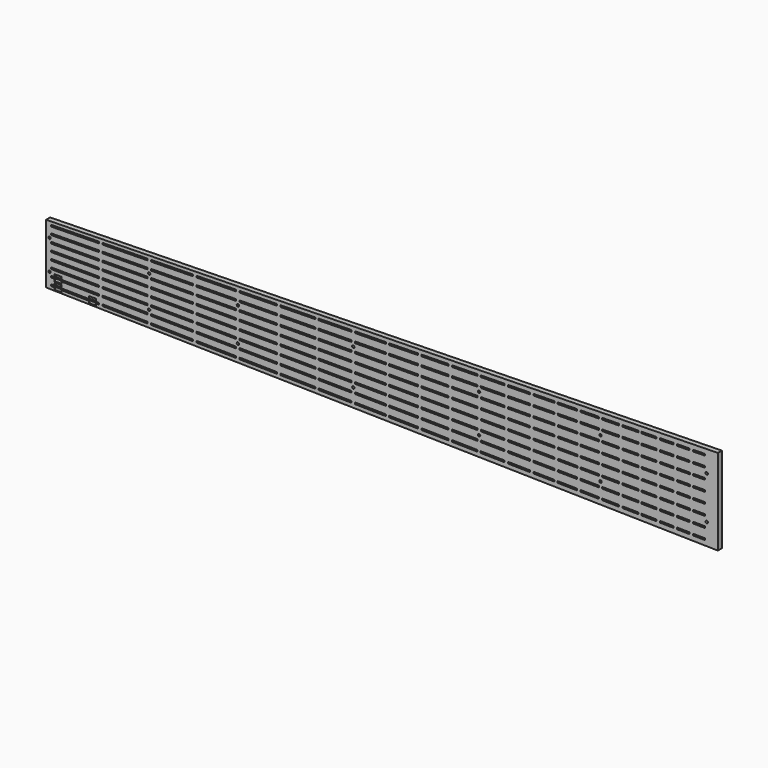
from build123d import *

# Parameters (mm, degrees)
F2_DEPTH  = 4.7625
F4_DEPTH  = 4.7635
F5_R      = 1.1303
F6_DEPTH  = 984
F8_DEPTH  = 4.7635
F9_W      = 6.5
F9_H      = 6.5
F10_DEPTH = 1


# Not quite as in the source:
# - an extrude ends at something that could not be found from the text; its depth is read off the source's solid


with BuildPart() as f2:
    # F1 (on Front) → F2 (new body)
    with BuildSketch(Plane.XZ):
        Polygon((0, 56.388), (0, 0), (635, -12.446), (635, 68.834), align=None)
    extrude(amount=F2_DEPTH)

    # F0 (on Front) → F4 (cut, through all)
    with BuildSketch(Plane.XZ):
        Polygon((4.7746291289, 4.2061348375), (4.7618279084, 3.4442423721), (4.749026688, 2.6823499068), (50.0380481272, 1.9214095194), (50.0508493476, 2.6833019848), (50.0636505681, 3.4451944501), align=None)
        Polygon((53.2382025071, 3.3918560315), (53.2254012866, 2.6299635662), (53.2126000661, 1.8680711009), (95.7808019259, 1.1528455786), (95.7936031464, 1.9147380439), (95.8064043669, 2.6766305093), align=None)
        Polygon((98.9809563058, 2.6232920907), (98.9681550853, 1.8613996253), (98.9553538649, 1.09950716), (138.9572987301, 0.4273995619), (138.9700999505, 1.1892920272), (138.982901171, 1.9511844925), align=None)
        Polygon((142.1574531099, 1.897846074), (142.1446518895, 1.1359536086), (142.131850669, 0.3740611433), (179.7022411275, -0.2571917865), (179.7150423479, 0.5047006789), (179.7278435684, 1.2665931442), align=None)
        Polygon((182.9023955073, 1.2132547257), (182.8895942869, 0.4513622603), (182.8767930664, -0.310530205), (218.1753725717, -0.9036124556), (218.1881737921, -0.1417199903), (218.2009750126, 0.6201724751), align=None)
        Polygon((221.3755269515, 0.5668340565), (221.3627257311, -0.1950584089), (221.3499245106, -0.9569508742), (254.4811739161, -1.5136179197), (254.4939751366, -0.7517254543), (254.506776357, 0.010167011), align=None)
        Polygon((257.681328296, -0.0431714076), (257.6685270755, -0.8050638729), (257.6557258551, -1.5669563382), (288.750030358, -2.0893988941), (288.7628315785, -1.3275064288), (288.775632799, -0.5656139634), align=None)
        Polygon((291.9501847379, -0.618952382), (291.9373835174, -1.3808448473), (291.924582297, -2.1427373127), (321.0950575321, -2.6328559335), (321.1078587526, -1.8709634681), (321.120659973, -1.1090710028), align=None)
        Polygon((324.295211912, -1.1624094214), (324.2824106915, -1.9243018867), (324.2696094711, -2.6861943521), (351.6250536824, -3.1458170521), (351.6378549029, -2.3839245867), (351.6506561233, -1.6220321214), align=None)
        Polygon((354.8252080623, -1.67537054), (354.8124068418, -2.4372630053), (354.7996056214, -3.1991554707), (380.441909228, -3.6299941998), (380.4547104484, -2.8681017344), (380.4675116689, -2.1062092691), align=None)
        Polygon((383.6420636078, -2.1595476876), (383.6292623874, -2.921440153), (383.6164611669, -3.6833326183), (407.6406067628, -4.086983262), (407.6534079833, -3.3250907967), (407.6662092037, -2.5631983313), align=None)
        Polygon((410.8407611427, -2.6165367499), (410.8279599222, -3.3784292152), (410.8151587017, -4.1403216806), (433.3135384465, -4.5183366002), (433.326339667, -3.7564441348), (433.3391408874, -2.9945516695), align=None)
        Polygon((436.5136928264, -3.0478900881), (436.5008916059, -3.8097825534), (436.4880903855, -4.5716750188), (457.5453251356, -4.9254760032), (457.558126356, -4.1635835378), (457.5709275765, -3.4016910725), align=None)
        Polygon((460.7454795155, -3.455029491), (460.732678295, -4.2169219564), (460.7198770745, -4.9788144217), (480.417133774, -5.3097652276), (480.4299349945, -4.5478727623), (480.4427362149, -3.7859802969), align=None)
        Polygon((483.6172881539, -3.8393187155), (483.6044869334, -4.6012111808), (483.591685713, -5.3631036462), (502.004950437, -5.672480982), (502.0177516575, -4.9105885166), (502.0305528779, -4.1486960513), align=None)
        Polygon((505.2051048169, -4.2020344698), (505.1923035964, -4.9639269352), (505.179502376, -5.7258194005), (522.3813072873, -6.0148419423), (522.3941085077, -5.252949477), (522.4069097282, -4.4910570116), align=None)
        Polygon((525.5814616672, -4.5443954302), (525.5686604467, -5.3062878956), (525.5558592262, -6.0681803609), (541.6135556188, -6.3379797367), (541.6263568392, -5.5760872713), (541.6391580597, -4.814194806), align=None)
        Polygon((544.8137099986, -4.8675332245), (544.8009087782, -5.6294256899), (544.7881075577, -6.3913181552), (559.7673197691, -6.6429969767), (559.7801209896, -5.8811045114), (559.79292221, -5.119212046), align=None)
        Polygon((562.967474149, -5.1725504646), (562.9546729285, -5.93444293), (562.9418717081, -6.6963353953), (576.901316251, -6.9308802099), (576.9141174715, -6.1689877446), (576.9269186919, -5.4070952792), align=None)
        Polygon((580.1014706309, -5.4604336978), (580.0886694104, -6.2223261632), (580.07586819, -6.9842186285), (593.0742615771, -7.2026159837), (593.0870627976, -6.4407235183), (593.099864018, -5.678831053), align=None)
        Polygon((596.274415957, -5.7321694715), (596.2616147365, -6.4940619369), (596.2488135161, -7.2559544022), (608.3388279132, -7.4590892889), (608.3516291337, -6.6971968236), (608.3644303541, -5.9353043582), align=None)
        Polygon((611.5389822931, -5.9886427768), (611.5261810726, -6.7505352421), (611.5133798522, -7.5124277075), (622.747687425, -7.7011851168), (622.7604886455, -6.9392926514), (622.773289866, -6.1774001861), align=None)
        Polygon((4.7713008369, 11.2775468317), (4.762157108, 10.5156016944), (4.7530133791, 9.7536565571), (50.0451657853, 9.210127709), (50.0543095142, 9.9720728463), (50.0634532431, 10.7340179835), align=None)
        Polygon((53.2382246484, 10.6959191131), (53.2290809195, 9.9339739759), (53.2199371906, 9.1720288386), (95.7910819189, 8.6611534655), (95.8002256478, 9.4230986028), (95.8093693767, 10.1850437401), align=None)
        Polygon((98.984140782, 10.1469448697), (98.9749970531, 9.3849997324), (98.9658533242, 8.6230545951), (138.9705636448, 8.1429777393), (138.9797073737, 8.9049228766), (138.9888511026, 9.6668680139), align=None)
        Polygon((142.1636225079, 9.6287691434), (142.154478779, 8.8668240062), (142.1453350501, 8.1048788689), (179.7183228632, 7.6539839191), (179.7274665921, 8.4159290563), (179.736610321, 9.1778741936), align=None)
        Polygon((182.9113817264, 9.1397753232), (182.9022379975, 8.3778301859), (182.8930942686, 7.6158850487), (218.1941140714, 7.1922548697), (218.2032578003, 7.9542000069), (218.2124015292, 8.7161451442), align=None)
        Polygon((221.3871729345, 8.6780462738), (221.3780292056, 7.9161011365), (221.3688854767, 7.1541559992), (254.5024253456, 6.7565366811), (254.5115690745, 7.5184818183), (254.5207128034, 8.2804269556), align=None)
        Polygon((257.6954842087, 8.2423280852), (257.6863404798, 7.4803829479), (257.6771967509, 6.7184378106), (288.7736508972, 6.3452645565), (288.7827946261, 7.1072096937), (288.791938355, 7.869154831), align=None)
        Polygon((291.9667097603, 7.8310559606), (291.9575660314, 7.0691108233), (291.9484223025, 6.307165686), (321.1209141808, 5.9570809569), (321.1300579097, 6.7190260942), (321.1392016386, 7.4809712315), align=None)
        Polygon((324.3139730439, 7.4428723611), (324.304829315, 6.6809272238), (324.2956855861, 5.9189820865), (351.6530209621, 5.5906801579), (351.662164691, 6.3526252952), (351.6713084198, 7.1145704325), align=None)
        Polygon((354.8460798252, 7.0764715621), (354.8369360963, 6.3145264248), (354.8277923674, 5.5525812875), (380.471868704, 5.2448393381), (380.4810124329, 6.0067844754), (380.4901561618, 6.7687296127), align=None)
        Polygon((383.6649275671, 6.7306307423), (383.6557838382, 5.968685605), (383.6466401093, 5.2067404677), (407.672446567, 4.9184185794), (407.6815902959, 5.6803637167), (407.6907340248, 6.4423088539), align=None)
        Polygon((410.8655054301, 6.4042099835), (410.8563617012, 5.6422648463), (410.8472179723, 4.880319709), (433.3471530981, 4.6103090521), (433.356296827, 5.3722541894), (433.3654405559, 6.1341993267), align=None)
        Polygon((436.5402119612, 6.0961004563), (436.5310682323, 5.334155319), (436.5219245034, 4.5722101817), (457.5806150038, 4.3194951929), (457.5897587327, 5.0814403301), (457.5989024616, 5.8433854674), align=None)
        Polygon((460.7736738669, 5.805286597), (460.764530138, 5.0433414597), (460.7553864091, 4.2813963224), (480.4540048395, 4.0450028897), (480.4631485684, 4.8069480269), (480.4722922973, 5.5688931642), align=None)
        Polygon((483.6470637027, 5.5307942938), (483.6379199738, 4.7688491565), (483.6287762449, 4.0069040193), (502.0433139336, 3.785920208), (502.0524576625, 4.5478653453), (502.0616013914, 5.3098104826), align=None)
        Polygon((505.2363727967, 5.2717116122), (505.2272290678, 4.5097664749), (505.2180853389, 3.7478213376), (522.421079463, 3.5413766649), (522.4302231919, 4.3033218021), (522.4393669208, 5.0652669394), align=None)
        Polygon((525.6141383261, 5.027168069), (525.6049945972, 4.2652229317), (525.5958508683, 3.5032777945), (541.6546573779, 3.3105639546), (541.6638011068, 4.0725090919), (541.6729448357, 4.8344542292), align=None)
        Polygon((544.8477162411, 4.7963553588), (544.8385725122, 4.0344102215), (544.8294287833, 3.2724650842), (559.8096765529, 3.0926944974), (559.8188202818, 3.8546396347), (559.8279640107, 4.616584772), align=None)
        Polygon((563.002735416, 4.5784859016), (562.9935916871, 3.8165407643), (562.9844479582, 3.054595627), (576.9448575598, 2.8870636166), (576.9540012887, 3.6490087539), (576.9631450176, 4.4109538911), align=None)
        Polygon((580.1379164229, 4.3728550207), (580.128772694, 3.6109098835), (580.1196289651, 2.8489647462), (593.1189209705, 2.6929666354), (593.1280646994, 3.4549117726), (593.1372084283, 4.2168569099), align=None)
        Polygon((596.3119798336, 4.1787580395), (596.3028361047, 3.4168129022), (596.2936923758, 2.654867765), (608.3845425922, 2.5097714173), (608.3936863211, 3.2717165546), (608.40283005, 4.0336616919), align=None)
        Polygon((611.5776014553, 3.9955628215), (611.5684577264, 3.2336176842), (611.5593139975, 2.4716725469), (622.7943982321, 2.336845826), (622.803541961, 3.0987909633), (622.8126856899, 3.8607361005), align=None)
        Polygon((4.7678627991, 18.3489412665), (4.7623765617, 17.5869610166), (4.7568903244, 16.8249807668), (50.0511299217, 16.4988634579), (50.056616159, 17.2608437078), (50.0621023963, 18.0228239576), align=None)
        Polygon((53.2370201042, 17.9999646354), (53.2315338668, 17.2379843855), (53.2260476295, 16.4760041356), (95.7991541571, 16.1694789118), (95.8046403944, 16.9314591617), (95.8101266318, 17.6934394115), align=None)
        Polygon((98.9850443396, 17.6705800893), (98.9795581022, 16.9085998394), (98.9740718649, 16.1466195896), (138.9806257162, 15.8585734761), (138.9861119535, 16.6205537259), (138.9915981909, 17.3825339758), align=None)
        Polygon((142.1665158987, 17.3596746536), (142.1610296613, 16.5976944037), (142.155543424, 15.8357141538), (179.7302627072, 15.5651771839), (179.7357489445, 16.3271574338), (179.7412351818, 17.0891376837), align=None)
        Polygon((182.9161528897, 17.0662783614), (182.9106666523, 16.3042981116), (182.905180415, 15.5423178617), (218.2078269891, 15.2881397543), (218.2133132264, 16.0501200042), (218.2187994637, 16.812100254), align=None)
        Polygon((221.3937171716, 16.7892409318), (221.3882309342, 16.0272606819), (221.3827446969, 15.265280432), (254.5178114535, 15.0267088411), (254.5232976908, 15.788689091), (254.5287839282, 16.5506693409), align=None)
        Polygon((257.703701636, 16.5278100186), (257.6982153986, 15.7658297688), (257.6927291613, 15.0038495189), (288.7906163205, 14.7799455664), (288.7961025579, 15.5419258162), (288.8015887952, 16.3039060661), align=None)
        Polygon((291.976506503, 16.2810467439), (291.9710202657, 15.519066494), (291.9655340283, 14.7570862441), (321.1393702579, 14.5470354066), (321.1448564953, 15.3090156565), (321.1503427326, 16.0709959064), align=None)
        Polygon((324.3252604404, 16.0481365841), (324.3197742031, 15.2861563343), (324.3142879658, 14.5241760844), (351.6728840454, 14.3271949272), (351.6783702828, 15.0891751771), (351.6838565201, 15.851155427), align=None)
        Polygon((354.8587742279, 15.8282961047), (354.8532879906, 15.0663158549), (354.8478017532, 14.304335605), (380.4930598417, 14.1196904354), (380.4985460791, 14.8816706853), (380.5040323164, 15.6436509351), align=None)
        Polygon((383.6789500242, 15.6207916129), (383.6734637869, 14.858811363), (383.6679775495, 14.0968311131), (407.6948911847, 13.9238379801), (407.700377422, 14.68581823), (407.7058636593, 15.4477984799), align=None)
        Polygon((410.8807813671, 15.4249391576), (410.8752951298, 14.6629589078), (410.8698088925, 13.9009786579), (433.3707808792, 13.7389722638), (433.3762671165, 14.5009525136), (433.3817533539, 15.2629327635), align=None)
        Polygon((436.5566710617, 15.2400734413), (436.5511848243, 14.4780931914), (436.545698587, 13.7161129415), (457.6053595317, 13.5644839482), (457.6108457691, 14.3264641981), (457.6163320064, 15.088444448), align=None)
        Polygon((460.7912497142, 15.0655851257), (460.7857634769, 14.3036048758), (460.7802772395, 13.541624626), (480.4798034382, 13.3997885663), (480.4852896756, 14.1617688162), (480.4907759129, 14.923749066), align=None)
        Polygon((483.6656936207, 14.9008897438), (483.6602073834, 14.1389094939), (483.6547211461, 13.376929244), (502.070107429, 13.2443389573), (502.0755936663, 14.0063192072), (502.0810799037, 14.768299457), align=None)
        Polygon((505.2559976115, 14.7454401348), (505.2505113741, 13.9834598849), (505.2450251368, 13.221479635), (522.4488120238, 13.0976128314), (522.4542982611, 13.8595930813), (522.4597844984, 14.6215733312), align=None)
        Polygon((525.6347022062, 14.5987140089), (525.6292159689, 13.836733759), (525.6237297316, 13.0747535092), (541.6832762766, 12.9591252053), (541.688762514, 13.7211054551), (541.6942487513, 14.483085705), align=None)
        Polygon((544.8691664591, 14.4602263828), (544.8636802218, 13.6982461329), (544.8581939844, 12.936265883), (559.8391320864, 12.828403531), (559.8446183238, 13.5903837808), (559.8501045611, 14.3523640307), align=None)
        Polygon((563.0250222689, 14.3295047085), (563.0195360316, 13.5675244586), (563.0140497943, 12.8055442087), (576.9751027312, 12.7050250024), (576.9805889685, 13.4670052523), (576.9860752058, 14.2289855022), align=None)
        Polygon((580.1609929136, 14.2061261799), (580.1555066763, 13.4441459301), (580.150020439, 12.6821656802), (593.1499114887, 12.5885668137), (593.155397726, 13.3505470636), (593.1608839634, 14.1125273135), align=None)
        Polygon((596.3358016712, 14.0896679912), (596.3303154338, 13.3276877413), (596.3248291965, 12.5657074915), (608.4162365936, 12.4786496829), (608.4217228309, 13.2406299328), (608.4272090683, 14.0026101826), align=None)
        Polygon((611.6021267761, 13.9797508604), (611.5966405388, 13.2177706105), (611.5911543014, 12.4557903606), (622.8267562806, 12.3748943281), (622.8322425179, 13.136874578), (622.8377287552, 13.8988548278), align=None)
        Polygon((4.7643150306, 25.4203181444), (4.7624862848, 24.6583203389), (4.760657539, 23.8963225333), (50.0559406958, 23.7876167637), (50.0577694415, 24.5496145693), (50.0595981873, 25.3116123748), align=None)
        Polygon((53.2345890439, 25.3039926007), (53.2327602981, 24.5419947952), (53.2309315523, 23.7799969896), (95.8050189457, 23.677821915), (95.8068476914, 24.4398197206), (95.8086764372, 25.2018175261), align=None)
        Polygon((98.9836672938, 25.194197752), (98.981838548, 24.4321999465), (98.9800098022, 23.6702021409), (138.987485387, 23.5741867697), (138.9893141328, 24.3361845753), (138.9911428786, 25.0981823809), align=None)
        Polygon((142.1661337351, 25.0905626068), (142.1643049893, 24.3285648012), (142.1624762435, 23.5665669957), (179.7380612318, 23.4763880057), (179.7398899776, 24.2383858113), (179.7417187234, 25.0003836168), align=None)
        Polygon((182.9167095799, 24.9927638428), (182.9148808341, 24.2307660372), (182.9130520883, 23.4687682316), (218.2165120199, 23.3840421958), (218.2183407657, 24.1460400014), (218.2201695115, 24.908037807), align=None)
        Polygon((221.395160368, 24.9004180329), (221.3933316223, 24.1384202273), (221.3915028765, 23.3764224217), (254.5273330505, 23.2968985581), (254.5291617963, 24.0588963637), (254.5309905421, 24.8208941692), align=None)
        Polygon((257.7059813986, 24.8132743952), (257.7041526528, 24.0512765896), (257.7023239071, 23.289278784), (288.800927548, 23.2146441332), (288.8027562938, 23.9766419387), (288.8045850396, 24.7386397443), align=None)
        Polygon((291.9795758961, 24.7310199702), (291.9777471503, 23.9690221647), (291.9759184045, 23.2070243591), (321.1504267866, 23.1370074133), (321.1522555324, 23.8990052188), (321.1540842781, 24.6610030244), align=None)
        Polygon((324.3290751347, 24.6533832503), (324.3272463889, 23.8913854448), (324.3254176431, 23.1293876392), (351.6846440529, 23.0637272535), (351.6864727986, 23.825725059), (351.6883015444, 24.5877228646), align=None)
        Polygon((354.8632924009, 24.5801030905), (354.8614636552, 23.818105285), (354.8596349094, 23.0561074794), (380.5054838534, 22.9945590895), (380.5073125992, 23.7565568951), (380.509141345, 24.5185547007), align=None)
        Polygon((383.6841322015, 24.5109349266), (383.6823034557, 23.748937121), (383.6804747099, 22.9869393154), (407.7079419146, 22.9292749378), (407.7097706604, 23.6912727433), (407.7115994062, 24.4532705489), align=None)
        Polygon((410.8865902627, 24.4456507748), (410.8847615169, 23.6836529693), (410.8829327712, 22.9216551637), (433.3844231704, 22.8676530323), (433.3862519162, 23.6296508379), (433.388080662, 24.3916486434), align=None)
        Polygon((436.5630715185, 24.3840288694), (436.5612427727, 23.6220310638), (436.559414027, 22.8600332582), (457.6195601771, 22.8094902605), (457.6213889229, 23.571488066), (457.6232176686, 24.3334858716), align=None)
        Polygon((460.7982085252, 24.3258660975), (460.7963797794, 23.5638682919), (460.7945510336, 22.8018704864), (480.4945311008, 22.7545917998), (480.4963598466, 23.5165896054), (480.4981885923, 24.278587411), align=None)
        Polygon((483.6731794489, 24.2709676369), (483.6713507031, 23.5089698313), (483.6695219573, 22.7469720257), (502.0853325227, 22.7027752635), (502.0871612685, 23.4647730691), (502.0889900143, 24.2267708746), align=None)
        Polygon((505.2639808708, 24.2191511005), (505.262152125, 23.457153295), (505.2603233792, 22.6951554894), (522.4645066339, 22.6538665549), (522.4663353797, 23.4158643604), (522.4681641255, 24.177862166), align=None)
        Polygon((525.643154982, 24.1702423919), (525.6413262362, 23.4082445863), (525.6394974904, 22.6462467808), (541.6994140404, 22.6077040128), (541.7012427862, 23.3697018184), (541.703071532, 24.1316996239), align=None)
        Polygon((544.8780623885, 24.1240798499), (544.8762336427, 23.3620820443), (544.8744048969, 22.6000842387), (559.8556881532, 22.5641301214), (559.857516899, 23.3261279269), (559.8593456448, 24.0881257325), align=None)
        Polygon((563.0343365013, 24.0805059584), (563.0325077555, 23.3185081529), (563.0306790097, 22.5565103473), (576.9920536032, 22.5230039452), (576.993882349, 23.2850017508), (576.9957110948, 24.0469995563), align=None)
        Polygon((580.1707019513, 24.0393797823), (580.1688732055, 23.2773819767), (580.1670444597, 22.5153841711), (593.1672350212, 22.484184549), (593.169063767, 23.2461823545), (593.1708925128, 24.0081801601), align=None)
        Polygon((596.3458833693, 24.000560386), (596.3440546235, 23.2385625804), (596.3422258778, 22.4765647749), (608.4339118556, 22.4475455054), (608.4357406014, 23.2095433109), (608.4375693472, 23.9715411165), align=None)
        Polygon((611.6125602037, 23.9639213424), (611.6107314579, 23.2019235368), (611.6089027122, 22.4399257313), (622.8447635547, 22.4129603871), (622.8465923004, 23.1749581927), (622.8484210462, 23.9369559982), align=None)
        Polygon((218.2133132264, 40.3378799958), (218.2078269891, 41.0998602457), (182.905180415, 40.8456821383), (182.9106666523, 40.0837018884), (182.9161528897, 39.3217216386), (218.2187994637, 39.575899746), align=None)
        Polygon((95.7936031464, 54.4732619561), (95.7808019259, 55.2351544214), (53.2126000661, 54.5199288991), (53.2254012866, 53.7580364338), (53.2382025071, 52.9961439685), (95.8064043669, 53.7113694907), align=None)
        Polygon((50.0508493476, 53.7046980152), (50.0380481272, 54.4665904806), (4.749026688, 53.7056500932), (4.7618279084, 52.9437576279), (4.7746291289, 52.1818651625), (50.0636505681, 52.9428055499), align=None)
        Polygon((182.9113817264, 47.2482246768), (218.2124015292, 47.6718548558), (218.2032578003, 48.4337999931), (218.1941140714, 49.1957451303), (182.8930942686, 48.7721149513), (182.9022379975, 48.0101698141), align=None)
        Polygon((324.3139730439, 48.9451276389), (351.6713084198, 49.2734295675), (351.662164691, 50.0353747048), (351.6530209621, 50.7973198421), (324.2956855861, 50.4690179135), (324.304829315, 49.7070727762), align=None)
        Polygon((354.8277923674, 50.8354187125), (354.8369360963, 50.0734735752), (354.8460798252, 49.3115284379), (380.4901561618, 49.6192703873), (380.4810124329, 50.3812155246), (380.471868704, 51.1431606619), align=None)
        Polygon((4.7568903244, 39.5630192332), (4.7623765617, 38.8010389834), (4.7678627991, 38.0390587335), (50.0621023963, 38.3651760424), (50.056616159, 39.1271562922), (50.0511299217, 39.8891365421), align=None)
        Polygon((98.9553538649, 55.28849284), (98.9681550853, 54.5266003747), (98.9809563058, 53.7647079093), (138.982901171, 54.4368155075), (138.9700999505, 55.1987079728), (138.9572987301, 55.9606004381), align=None)
        Polygon((324.3142879658, 41.8638239156), (324.3197742031, 41.1018436657), (324.3252604404, 40.3398634159), (351.6838565201, 40.536844573), (351.6783702828, 41.2988248229), (351.6728840454, 42.0608050728), align=None)
        Polygon((321.1300579097, 49.6689739058), (321.1209141808, 50.4309190431), (291.9484223025, 50.080834314), (291.9575660314, 49.3188891767), (291.9667097603, 48.5569440394), (321.1392016386, 48.9070287685), align=None)
        Polygon((541.6638011068, 52.3154909081), (541.6546573779, 53.0774360454), (525.5958508683, 52.8847222055), (525.6049945972, 52.1227770683), (525.6141383261, 51.360831931), (541.6729448357, 51.5535457708), align=None)
        Polygon((53.2382246484, 45.6920808869), (95.8093693767, 46.2029562599), (95.8002256478, 46.9649013972), (95.7910819189, 47.7268465345), (53.2199371906, 47.2159711614), (53.2290809195, 46.4540260241), align=None)
        Polygon((410.8698088925, 42.4870213421), (410.8752951298, 41.7250410922), (410.8807813671, 40.9630608424), (433.3817533539, 41.1250672365), (433.3762671165, 41.8870474864), (433.3707808792, 42.6490277362), align=None)
        Polygon((522.4302231919, 52.0846781979), (522.421079463, 52.8466233351), (505.2180853389, 52.6401786624), (505.2272290678, 51.8782335251), (505.2363727967, 51.1162883878), (522.4393669208, 51.3227330606), align=None)
        Polygon((257.6954842087, 48.1456719148), (288.791938355, 48.518845169), (288.7827946261, 49.2807903063), (288.7736508972, 50.0427354435), (257.6771967509, 49.6695621894), (257.6863404798, 48.9076170521), align=None)
        Polygon((544.8294287833, 53.1155349158), (544.8385725122, 52.3535897785), (544.8477162411, 51.5916446412), (559.8279640107, 51.771415228), (559.8188202818, 52.5333603653), (559.8096765529, 53.2953055026), align=None)
        Polygon((608.3936863211, 53.1162834454), (608.3845425922, 53.8782285827), (596.2936923758, 53.733132235), (596.3028361047, 52.9711870978), (596.3119798336, 52.2092419605), (608.40283005, 52.3543383081), align=None)
        Polygon((611.5911543014, 43.9322096394), (611.5966405388, 43.1702293895), (611.6021267761, 42.4082491396), (622.8377287552, 42.4891451722), (622.8322425179, 43.251125422), (622.8267562806, 44.0131056719), align=None)
        Polygon((182.9130520883, 32.9192317684), (182.9148808341, 32.1572339628), (182.9167095799, 31.3952361572), (218.2201695115, 31.479962193), (218.2183407657, 32.2419599986), (218.2165120199, 33.0039578042), align=None)
        Polygon((460.7912497142, 41.3224148743), (480.4907759129, 41.464250934), (480.4852896756, 42.2262311838), (480.4798034382, 42.9882114337), (460.7802772395, 42.846375374), (460.7857634769, 42.0843951242), align=None)
        Polygon((179.7274665921, 47.9720709437), (179.7183228632, 48.7340160809), (142.1453350501, 48.2831211311), (142.154478779, 47.5211759938), (142.1636225079, 46.7592308566), (179.736610321, 47.2101258064), align=None)
        Polygon((4.7713008369, 45.1104531683), (50.0634532431, 45.6539820165), (50.0543095142, 46.4159271537), (50.0451657853, 47.177872291), (4.7530133791, 46.6343434429), (4.762157108, 45.8723983056), align=None)
        Polygon((179.7398899776, 32.1496141887), (179.7380612318, 32.9116119943), (142.1624762435, 32.8214330043), (142.1643049893, 32.0594351988), (142.1661337351, 31.2974373932), (179.7417187234, 31.3876163832), align=None)
        Polygon((480.4631485684, 51.5810519731), (480.4540048395, 52.3429971103), (460.7553864091, 52.1066036776), (460.764530138, 51.3446585403), (460.7736738669, 50.582713403), (480.4722922973, 50.8191068358), align=None)
        Polygon((98.9850443396, 38.7174199107), (138.9915981909, 39.0054660242), (138.9861119535, 39.7674462741), (138.9806257162, 40.5294265239), (98.9740718649, 40.2413804104), (98.9795581022, 39.4794001606), align=None)
        Polygon((291.9655340283, 41.6309137559), (291.9710202657, 40.868933506), (291.976506503, 40.1069532561), (321.1503427326, 40.3170040936), (321.1448564953, 41.0789843435), (321.1393702579, 41.8409645934), align=None)
        Polygon((257.6927291613, 41.3841504811), (257.6982153986, 40.6221702312), (257.703701636, 39.8601899814), (288.8015887952, 40.0840939339), (288.7961025579, 40.8460741838), (288.7906163205, 41.6080544336), align=None)
        Polygon((221.3827446969, 41.122719568), (221.3882309342, 40.3607393181), (221.3937171716, 39.5987590682), (254.5287839282, 39.8373306591), (254.5232976908, 40.599310909), (254.5178114535, 41.3612911589), align=None)
        Polygon((608.4217228309, 43.1473700672), (608.4162365936, 43.9093503171), (596.3248291965, 43.8222925085), (596.3303154338, 43.0603122587), (596.3358016712, 42.2983320088), (608.4272090683, 42.3853898174), align=None)
        Polygon((53.2260476295, 39.9119958644), (53.2315338668, 39.1500156145), (53.2370201042, 38.3880353646), (95.8101266318, 38.6945605885), (95.8046403944, 39.4565408383), (95.7991541571, 40.2185210882), align=None)
        Polygon((580.07586819, 63.3722186285), (580.0886694104, 62.6103261632), (580.1014706309, 61.8484336978), (593.099864018, 62.066831053), (593.0870627976, 62.8287235183), (593.0742615771, 63.5906159837), align=None)
        Polygon((182.9023955073, 55.1747452743), (218.2009750126, 55.7678275249), (218.1881737921, 56.5297199903), (218.1753725717, 57.2916124556), (182.8767930664, 56.698530205), (182.8895942869, 55.9366377397), align=None)
        Polygon((53.2345890439, 31.0840073993), (95.8086764372, 31.1861824739), (95.8068476914, 31.9481802794), (95.8050189457, 32.710178085), (53.2309315523, 32.6080030104), (53.2327602981, 31.8460052048), align=None)
        Polygon((142.155543424, 40.5522858462), (142.1610296613, 39.7903055963), (142.1665158987, 39.0283253464), (179.7412351818, 39.2988623163), (179.7357489445, 40.0608425662), (179.7302627072, 40.8228228161), align=None)
        Polygon((576.9805889685, 42.9209947477), (576.9751027312, 43.6829749976), (563.0140497943, 43.5824557913), (563.0195360316, 42.8204755414), (563.0250222689, 42.0584952915), (576.9860752058, 42.1590144978), align=None)
        Polygon((502.0524576625, 51.8401346547), (502.0433139336, 52.602079792), (483.6287762449, 52.3810959807), (483.6379199738, 51.6191508435), (483.6470637027, 50.8572057062), (502.0616013914, 51.0781895174), align=None)
        Polygon((436.5219245034, 51.8157898183), (436.5310682323, 51.053844681), (436.5402119612, 50.2918995437), (457.5989024616, 50.5446145326), (457.5897587327, 51.3065596699), (457.5806150038, 52.0685048071), align=None)
        Polygon((410.8655054301, 49.9837900165), (433.3654405559, 50.2538006733), (433.356296827, 51.0157458106), (433.3471530981, 51.7776909479), (410.8472179723, 51.507680291), (410.8563617012, 50.7457351537), align=None)
        Polygon((576.9141174715, 62.5569877446), (576.901316251, 63.3188802099), (562.9418717081, 63.0843353953), (562.9546729285, 62.32244293), (562.967474149, 61.5605504646), (576.9269186919, 61.7950952792), align=None)
        Polygon((4.7643150306, 30.9676818556), (50.0595981873, 31.0763876252), (50.0577694415, 31.8383854307), (50.0559406958, 32.6003832363), (4.760657539, 32.4916774667), (4.7624862848, 31.7296796611), align=None)
        Polygon((457.6108457691, 42.0615358019), (457.6053595317, 42.8235160518), (436.545698587, 42.6718870585), (436.5511848243, 41.9099068086), (436.5566710617, 41.1479265587), (457.6163320064, 41.299555552), align=None)
        Polygon((138.9893141328, 32.0518154247), (138.987485387, 32.8138132303), (98.9800098022, 32.7177978591), (98.981838548, 31.9558000535), (98.9836672938, 31.193802248), (138.9911428786, 31.2898176191), align=None)
        Polygon((383.6164611669, 60.0713326183), (383.6292623874, 59.309440153), (383.6420636078, 58.5475476876), (407.6662092037, 58.9511983313), (407.6534079833, 59.7130907967), (407.6406067628, 60.474983262), align=None)
        Polygon((291.924582297, 58.5307373127), (291.9373835174, 57.7688448473), (291.9501847379, 57.006952382), (321.120659973, 57.4970710028), (321.1078587526, 58.2589634681), (321.0950575321, 59.0208559335), align=None)
        Polygon((383.6466401093, 51.1812595323), (383.6557838382, 50.419314395), (383.6649275671, 49.6573692577), (407.6907340248, 49.9456911461), (407.6815902959, 50.7076362833), (407.672446567, 51.4695814206), align=None)
        Polygon((98.9658533242, 47.7649454049), (98.9749970531, 47.0030002676), (98.984140782, 46.2410551303), (138.9888511026, 46.7211319862), (138.9797073737, 47.4830771234), (138.9705636448, 48.2450222607), align=None)
        Polygon((611.5593139975, 53.9163274531), (611.5684577264, 53.1543823158), (611.5776014553, 52.3924371785), (622.8126856899, 52.5272638995), (622.803541961, 53.2892090367), (622.7943982321, 54.051154174), align=None)
        Polygon((608.3516291337, 63.0851968236), (608.3388279132, 63.8470892889), (596.2488135161, 63.6439544022), (596.2616147365, 62.8820619369), (596.274415957, 62.1201694715), (608.3644303541, 62.3233043582), align=None)
        Polygon((522.3941085077, 61.640949477), (522.3813072873, 62.4028419423), (505.179502376, 62.1138194005), (505.1923035964, 61.3519269352), (505.2051048169, 60.5900344698), (522.4069097282, 60.8790570116), align=None)
        Polygon((525.6237297316, 43.3132464908), (525.6292159689, 42.551266241), (525.6347022062, 41.7892859911), (541.6942487513, 41.904914295), (541.688762514, 42.6668945449), (541.6832762766, 43.4288747947), align=None)
        Polygon((580.1196289651, 53.5390352538), (580.128772694, 52.7770901165), (580.1379164229, 52.0151449793), (593.1372084283, 52.1711430901), (593.1280646994, 52.9330882274), (593.1189209705, 53.6950333646), align=None)
        Polygon((576.9540012887, 52.7389912461), (576.9448575598, 53.5009363834), (562.9844479582, 53.333404373), (562.9935916871, 52.5714592357), (563.002735416, 51.8095140984), (576.9631450176, 51.9770461089), align=None)
        Polygon((522.4542982611, 42.5284069187), (522.4488120238, 43.2903871686), (505.2450251368, 43.166520365), (505.2505113741, 42.4045401151), (505.2559976115, 41.6425598652), (522.4597844984, 41.7664266688), align=None)
        Polygon((436.4880903855, 60.9596750188), (436.5008916059, 60.1977825534), (436.5136928264, 59.4358900881), (457.5709275765, 59.7896910725), (457.558126356, 60.5515835378), (457.5453251356, 61.3134760032), align=None)
        Polygon((383.6789500242, 40.7672083871), (407.7058636593, 40.9402015201), (407.700377422, 41.70218177), (407.6948911846, 42.4641620199), (383.6679775495, 42.2911688869), (383.6734637869, 41.529188637), align=None)
        Polygon((179.7150423479, 55.8832993211), (179.7022411275, 56.6451917865), (142.131850669, 56.0139388567), (142.1446518895, 55.2520463914), (142.1574531099, 54.490153926), (179.7278435684, 55.1214068558), align=None)
        Polygon((354.8252080623, 58.06337054), (380.4675116689, 58.4942092691), (380.4547104484, 59.2561017344), (380.441909228, 60.0179941998), (354.7996056214, 59.5871554707), (354.8124068418, 58.8252630053), align=None)
        Polygon((291.9759184045, 33.1809756409), (291.9777471503, 32.4189778353), (291.9795758961, 31.6569800298), (321.1540842781, 31.7269969756), (321.1522555324, 32.4889947812), (321.1504267866, 33.2509925867), align=None)
        Polygon((483.6656936207, 41.4871102562), (502.0810799037, 41.619700543), (502.0755936663, 42.3816807928), (502.070107429, 43.1436610427), (483.6547211461, 43.011070756), (483.6602073834, 42.2490905061), align=None)
        Polygon((221.3688854767, 49.2338440008), (221.3780292056, 48.4718988635), (221.3871729345, 47.7099537262), (254.5207128034, 48.1075730444), (254.5115690745, 48.8695181817), (254.5024253456, 49.6314633189), align=None)
        Polygon((257.6557258551, 57.9549563382), (257.6685270755, 57.1930638729), (257.681328296, 56.4311714076), (288.775632799, 56.9536139634), (288.7628315785, 57.7155064288), (288.750030358, 58.4773988941), align=None)
        Polygon((354.8478017532, 42.083664395), (354.8532879906, 41.3216841451), (354.8587742279, 40.5597038953), (380.5040323164, 40.7443490649), (380.4985460791, 41.5063293147), (380.4930598417, 42.2683095646), align=None)
        Polygon((483.6172881539, 60.2273187155), (502.0305528779, 60.5366960513), (502.0177516575, 61.2985885166), (502.004950437, 62.060480982), (483.591685713, 61.7511036462), (483.6044869334, 60.9892111808), align=None)
        Polygon((324.2696094711, 59.0741943521), (324.2824106915, 58.3123018867), (324.295211912, 57.5504094214), (351.6506561233, 58.0100321214), (351.6378549029, 58.7719245867), (351.6250536824, 59.5338170521), align=None)
        Polygon((580.150020439, 43.7058343198), (580.1555066763, 42.9438540699), (580.1609929136, 42.1818738201), (593.1608839634, 42.2754726865), (593.155397726, 43.0374529364), (593.1499114887, 43.7994331863), align=None)
        Polygon((611.5133798522, 63.9004277075), (611.5261810726, 63.1385352421), (611.5389822931, 62.3766427768), (622.773289866, 62.5654001861), (622.7604886455, 63.3272926514), (622.747687425, 64.0891851168), align=None)
        Polygon((559.8446183238, 42.7976162192), (559.8391320864, 43.559596469), (544.8581939844, 43.451734117), (544.8636802218, 42.6897538671), (544.8691664591, 41.9277736172), (559.8501045611, 42.0356359693), align=None)
        Polygon((460.7454795155, 59.843029491), (480.4427362149, 60.1739802969), (480.4299349945, 60.9358727623), (480.417133774, 61.6977652276), (460.7198770745, 61.3668144217), (460.732678295, 60.6049219564), align=None)
        Polygon((525.5558592262, 62.4561803609), (525.5686604467, 61.6942878956), (525.5814616672, 60.9323954302), (541.6391580597, 61.202194806), (541.6263568392, 61.9640872713), (541.6135556188, 62.7259797367), align=None)
        Polygon((433.326339667, 60.1444441348), (433.3135384465, 60.9063366002), (410.8151587017, 60.5283216806), (410.8279599222, 59.7664292152), (410.8407611427, 59.0045367499), (433.3391408874, 59.3825516695), align=None)
        Polygon((544.7881075577, 62.7793181552), (544.8009087782, 62.0174256899), (544.8137099986, 61.2555332245), (559.79292221, 61.507212046), (559.7801209896, 62.2691045114), (559.7673197691, 63.0309969767), align=None)
        Polygon((221.3915028765, 33.0115775783), (221.3933316223, 32.2495797727), (221.395160368, 31.4875819671), (254.5309905421, 31.5671058308), (254.5291617963, 32.3291036363), (254.5273330505, 33.0911014419), align=None)
        Polygon((257.7059813986, 31.5747256048), (288.8045850396, 31.6493602557), (288.8027562938, 32.4113580613), (288.800927548, 33.1733558668), (257.7023239071, 33.098721216), (257.7041526528, 32.3367234104), align=None)
        Polygon((254.4939751366, 57.1397254543), (254.4811739161, 57.9016179197), (221.3499245106, 57.3449508742), (221.3627257311, 56.5830584089), (221.3755269515, 55.8211659435), (254.506776357, 56.377832989), align=None)
        Polygon((407.7097706604, 32.6967272567), (407.7079419146, 33.4587250622), (383.6804747099, 33.4010606846), (383.6823034557, 32.639062879), (383.6841322015, 31.8770650734), (407.7115994062, 31.9347294511), align=None)
        Polygon((324.3254176431, 33.2586123608), (324.3272463889, 32.4966145552), (324.3290751347, 31.7346167497), (351.6883015444, 31.8002771354), (351.6864727986, 32.562274941), (351.6846440529, 33.3242727465), align=None)
        Polygon((354.8596349094, 33.3318925206), (354.8614636552, 32.569894715), (354.8632924009, 31.8078969095), (380.509141345, 31.8694452993), (380.5073125992, 32.6314431049), (380.5054838534, 33.3934409105), align=None)
        Polygon((410.8829327712, 33.4663448363), (410.8847615169, 32.7043470307), (410.8865902627, 31.9423492252), (433.388080662, 31.9963513566), (433.3862519162, 32.7583491621), (433.3844231704, 33.5203469677), align=None)
        Polygon((480.4945311008, 33.6334082002), (460.7945510336, 33.5861295136), (460.7963797794, 32.8241317081), (460.7982085252, 32.0621339025), (480.4981885923, 32.109412589), (480.4963598466, 32.8714103946), align=None)
        Polygon((522.4645066339, 33.7341334451), (505.2603233792, 33.6928445106), (505.262152125, 32.930846705), (505.2639808708, 32.1688488995), (522.4681641255, 32.210137834), (522.4663353797, 32.9721356396), align=None)
        Polygon((483.6713507031, 32.8790301687), (483.6731794489, 32.1170323631), (502.0889900143, 32.1612291254), (502.0871612685, 32.9232269309), (502.0853325227, 33.6852247365), (483.6695219573, 33.6410279743), align=None)
        Polygon((436.559414027, 33.5279667418), (436.5612427727, 32.7659689362), (436.5630715185, 32.0039711306), (457.6232176686, 32.0545141284), (457.6213889229, 32.816511934), (457.6195601771, 33.5785097395), align=None)
        Polygon((559.8556881532, 33.8238698786), (544.8744048969, 33.7879157613), (544.8762336427, 33.0259179557), (544.8780623885, 32.2639201501), (559.8593456448, 32.2998742675), (559.857516899, 33.0618720731), align=None)
        Polygon((541.6994140404, 33.7802959872), (525.6394974904, 33.7417532192), (525.6413262362, 32.9797554137), (525.643154982, 32.2177576081), (541.703071532, 32.2563003761), (541.7012427862, 33.0182981816), align=None)
        Polygon((611.6125602037, 32.4240786576), (622.8484210462, 32.4510440018), (622.8465923004, 33.2130418073), (622.8447635547, 33.9750396129), (611.6089027122, 33.9480742687), (611.6107314579, 33.1860764632), align=None)
        Polygon((608.4357406014, 33.1784566891), (608.4339118556, 33.9404544946), (596.3422258778, 33.9114352251), (596.3440546235, 33.1494374196), (596.3458833693, 32.387439614), (608.4375693472, 32.4164588835), align=None)
        Polygon((563.0306790097, 33.8314896527), (563.0325077555, 33.0694918471), (563.0343365013, 32.3074940416), (576.9957110948, 32.3410004437), (576.993882349, 33.1029982492), (576.9920536032, 33.8649960548), align=None)
        Polygon((580.1670444597, 33.8726158289), (580.1688732055, 33.1106180233), (580.1707019513, 32.3486202177), (593.1708925128, 32.3798198399), (593.169063767, 33.1418176455), (593.1672350212, 33.903815451), align=None)
    extrude(amount=F4_DEPTH, mode=Mode.SUBTRACT)

    # F5 (on face) → F6 (cut, through all)
    with BuildSketch(Plane.XZ.offset(4.7625)):
        with Locations((97.3946236, 13.1425326887)):
            Circle(F5_R)
        with Locations((3.175, 14.065885)):
            Circle(F5_R)
        with Locations((181.3279076, 12.3199865055)):
            Circle(F5_R)
        with Locations((290.391088, 11.2511673376)):
            Circle(F5_R)
        with Locations((409.2984448, 10.085875241)):
            Circle(F5_R)
        with Locations((524.05534, 8.961257668)):
            Circle(F5_R)
        with Locations((624.435886, 7.9775283172)):
            Circle(F5_R)
        with Locations((97.3946236, 43.2454673113)):
            Circle(F5_R)
        with Locations((3.175, 42.322115)):
            Circle(F5_R)
        with Locations((181.3279076, 44.0680134945)):
            Circle(F5_R)
        with Locations((290.391088, 45.1368326624)):
            Circle(F5_R)
        with Locations((409.2984448, 46.302124759)):
            Circle(F5_R)
        with Locations((524.05534, 47.426742332)):
            Circle(F5_R)
        with Locations((624.435886, 48.4104716828)):
            Circle(F5_R)
    extrude(amount=F6_DEPTH, mode=Mode.SUBTRACT)

    # F5 (on face) → F8 (cut, through all)
    with BuildSketch(Plane.XZ.offset(4.7625)):
        with Locations((97.3946236, 13.1425326887)):
            Circle(F5_R)
        with Locations((3.175, 14.065885)):
            Circle(F5_R)
        with Locations((181.3279076, 12.3199865055)):
            Circle(F5_R)
        with Locations((290.391088, 11.2511673376)):
            Circle(F5_R)
        with Locations((409.2984448, 10.085875241)):
            Circle(F5_R)
        with Locations((524.05534, 8.961257668)):
            Circle(F5_R)
        with Locations((624.435886, 7.9775283172)):
            Circle(F5_R)
        with Locations((97.3946236, 43.2454673113)):
            Circle(F5_R)
        with Locations((3.175, 42.322115)):
            Circle(F5_R)
        with Locations((181.3279076, 44.0680134945)):
            Circle(F5_R)
        with Locations((290.391088, 45.1368326624)):
            Circle(F5_R)
        with Locations((409.2984448, 46.302124759)):
            Circle(F5_R)
        with Locations((524.05534, 47.426742332)):
            Circle(F5_R)
        with Locations((624.435886, 48.4104716828)):
            Circle(F5_R)
    extrude(amount=-F8_DEPTH, mode=Mode.SUBTRACT)

    # F9 (on face) → F10 (cut)
    with BuildSketch(Plane.XZ.offset(4.7625)):
        with Locations((11.1125, 3.3375391861)):
            Rectangle(F9_W, F9_H)
        with Locations((11.1125, 10.4393943522)):
            Rectangle(F9_W, F9_H)
        with Locations((43.7079136, 2.7900902703)):
            Rectangle(F9_W, F9_H)
    extrude(amount=-F10_DEPTH, mode=Mode.SUBTRACT)


solid = f2.part
